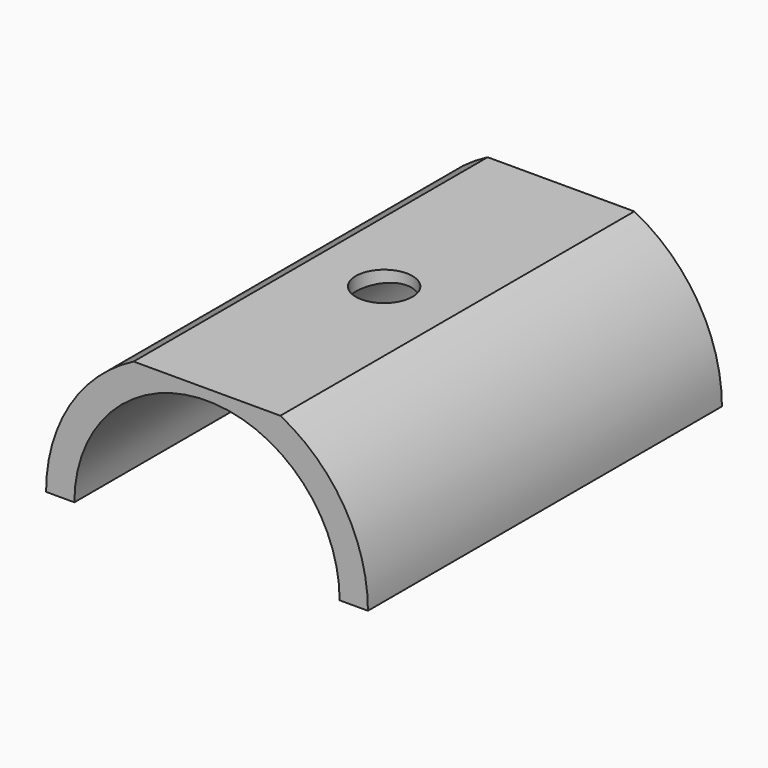
from build123d import *

# Parameters (mm, degrees)
F1_DEPTH = 125.1
F2_W     = 44
F2_H     = 8.367
F3_DEPTH = 125.1
F4_R     = 8
F5_DEPTH = 4


with BuildPart() as f1:
    # F0 (on Front) → F1 (new body)
    with BuildSketch(Plane.XZ):
        with BuildLine():
            ThreePointArc((-37.5, 0), (0, 37.5), (37.5, 0))
            Line((37.5, 0), (45.5, 0))
            ThreePointArc((45.5, 0), (0, 45.5), (-45.5, 0))
            Line((-45.5, 0), (-37.5, 0))
        make_face()
    extrude(amount=F1_DEPTH)

    # F2 (on Front) → F3 (cut)
    with BuildSketch(Plane.XZ):
        with Locations((0, 44.6835)):
            Rectangle(F2_W, F2_H)
    extrude(amount=F3_DEPTH, mode=Mode.SUBTRACT)

    # F4 (on face) → F5 (cut)
    with BuildSketch(Plane.XY.offset(40.5)):
        with Locations((0, -62.5)):
            Circle(F4_R)
    extrude(amount=-F5_DEPTH, mode=Mode.SUBTRACT)


solid = f1.part
